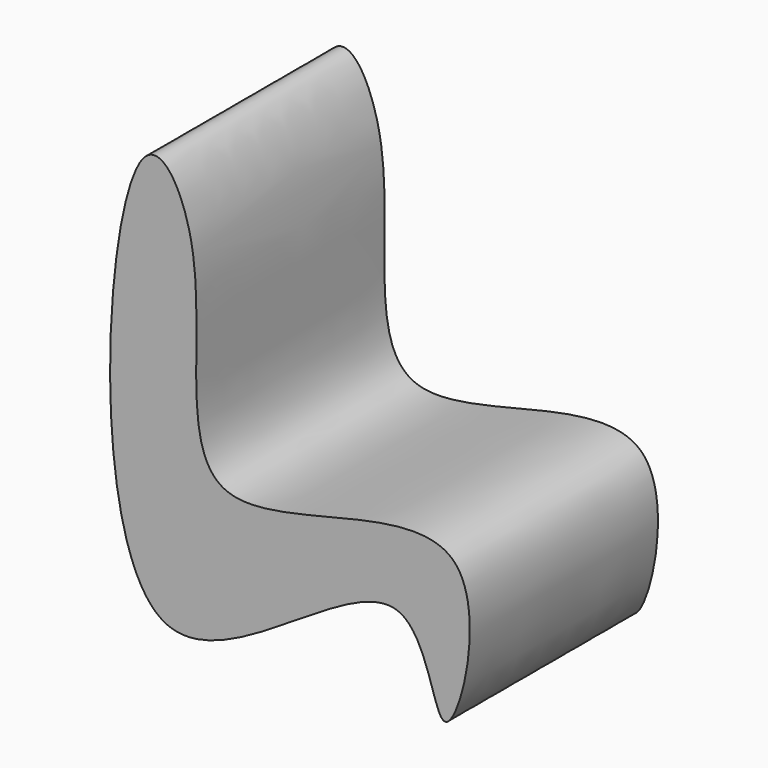
from build123d import *

# Parameters (mm, degrees)
F1_DEPTH = 60


# Not quite as in the source:
# - a feature of the source that left no trace in its solid (it failed there, or was rolled back) is left out
# - the program builds the solid bodies; features that only make, move or delete a surface that nothing else refers to are left out


with BuildPart() as f1:
    # F0 (on Front) → F1 (new body)
    with BuildSketch(Plane.XZ):
        with BuildLine():
            add(Edge.make_bspline(
                [(-36.3768599927, 34.6582718194), (-33.4418297724, 15.1140646105), (-46.8030180002, -39.0381180133), (47.1328492094, 13.2939671139), (26.2556378301, -72.0288161706), (21.934250444, -2.1057858824), (-67.2264525261, -103.5924696147), (-56.8944583898, 78.6498378435), (-38.2762900885, 47.3064739102), (-36.3768599927, 34.6582718194)],
                knots=[0, 0, 0, 0, 0.1477453621, 0.3046700823, 0.4296216232, 0.531251089, 0.6952959326, 0.9043853159, 1, 1, 1, 1], degree=3))
        make_face()
    extrude(amount=F1_DEPTH)


solid = f1.part
